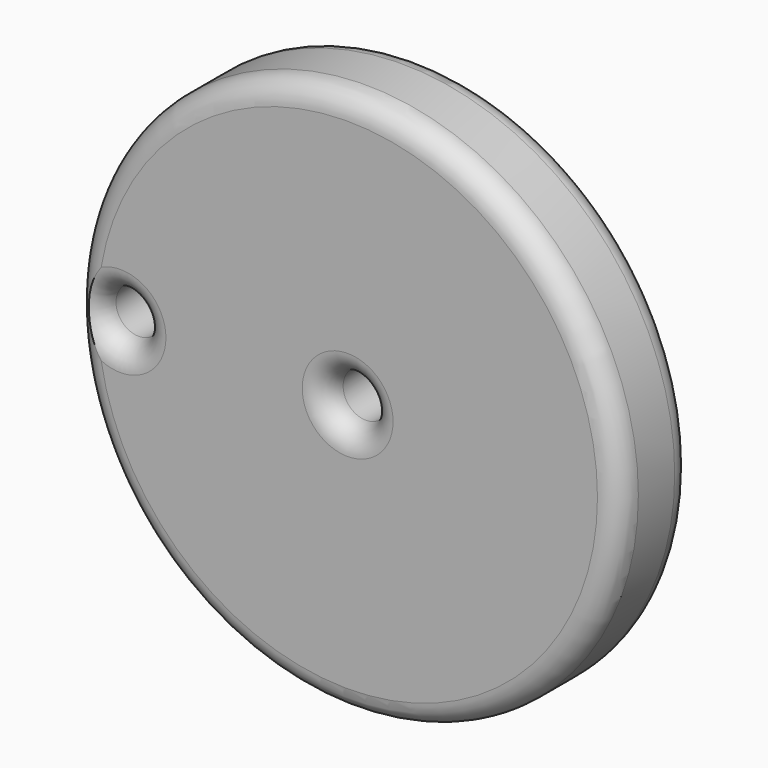
from build123d import *

# Parameters (mm, degrees)
F0_R     = 152.4
F1_DEPTH = 50.8
F2_R     = 12.7
F3_DEPTH = 50.801


# Not quite as in the source:
# - a fillet or chamfer that OpenCascade refuses, or shapes differently, is made with other operations: its cross-section is extruded or revolved along the edge and cut away or added


with BuildPart() as f1:
    # F0 (on Front) → F1 (new body)
    with BuildSketch(Plane.XZ):
        Circle(F0_R)
    extrude(amount=F1_DEPTH)

    # F2 (on face) → F3 (cut, through all)
    with BuildSketch(Plane.XZ.offset(50.8)):
        Circle(F2_R)
        with Locations((-127, 0)):
            Circle(F2_R)
    extrude(amount=-F3_DEPTH, mode=Mode.SUBTRACT)

    # F4: fillet of radius 12.7 on 6 edges, made by hand

    # F4_s1 → F4_t2 (revolve, cut)
    with BuildSketch(Plane.XY):
        with BuildLine():
            ThreePointArc((152.4, -38.1), (148.6802561211, -47.0802561211), (139.7, -50.8))
            Line((139.7, -50.8), (152.4, -50.8))
            Line((152.4, -50.8), (152.4, -38.1))
        make_face()
    revolve(axis=Axis((0, -50.8, 0), (0, -1, 0)), mode=Mode.SUBTRACT)

    # F4_s3 → F4_t4 (revolve, cut)
    with BuildSketch(Plane.XY):
        with BuildLine():
            ThreePointArc((-101.6, -50.8), (-110.5802561211, -47.0802561211), (-114.3, -38.1))
            Line((-114.3, -38.1), (-114.3, -50.8))
            Line((-114.3, -50.8), (-101.6, -50.8))
        make_face()
    revolve(axis=Axis((-127, -50.8, 0), (0, -1, 0)), mode=Mode.SUBTRACT)

    # F4_s5 → F4_t6 (revolve, cut)
    with BuildSketch(Plane.XY):
        with BuildLine():
            ThreePointArc((25.4, -50.8), (16.4197438789, -47.0802561211), (12.7, -38.1))
            Line((12.7, -38.1), (12.7, -50.8))
            Line((12.7, -50.8), (25.4, -50.8))
        make_face()
    revolve(axis=Axis((0, -50.8, 0), (0, -1, 0)), mode=Mode.SUBTRACT)

    # F4_s7 → F4_t8 (revolve, cut)
    with BuildSketch(Plane.XY):
        with BuildLine():
            ThreePointArc((152.4, -12.7), (148.6802561211, -3.7197438789), (139.7, 0))
            Line((139.7, 0), (152.4, 0))
            Line((152.4, 0), (152.4, -12.7))
        make_face()
    revolve(axis=Axis((0, 0, 0), (0, -1, 0)), mode=Mode.SUBTRACT)

    # F4_s9 → F4_t10 (revolve, cut)
    with BuildSketch(Plane.XY):
        with BuildLine():
            ThreePointArc((-101.6, 0), (-110.5802561211, -3.7197438789), (-114.3, -12.7))
            Line((-114.3, -12.7), (-114.3, 0))
            Line((-114.3, 0), (-101.6, 0))
        make_face()
    revolve(axis=Axis((-127, 0, 0), (0, -1, 0)), mode=Mode.SUBTRACT)

    # F4_s11 → F4_t12 (revolve, cut)
    with BuildSketch(Plane.XY):
        with BuildLine():
            ThreePointArc((25.4, 0), (16.4197438789, -3.7197438789), (12.7, -12.7))
            Line((12.7, -12.7), (12.7, 0))
            Line((12.7, 0), (25.4, 0))
        make_face()
    revolve(axis=Axis((0, 0, 0), (0, -1, 0)), mode=Mode.SUBTRACT)


solid = f1.part
